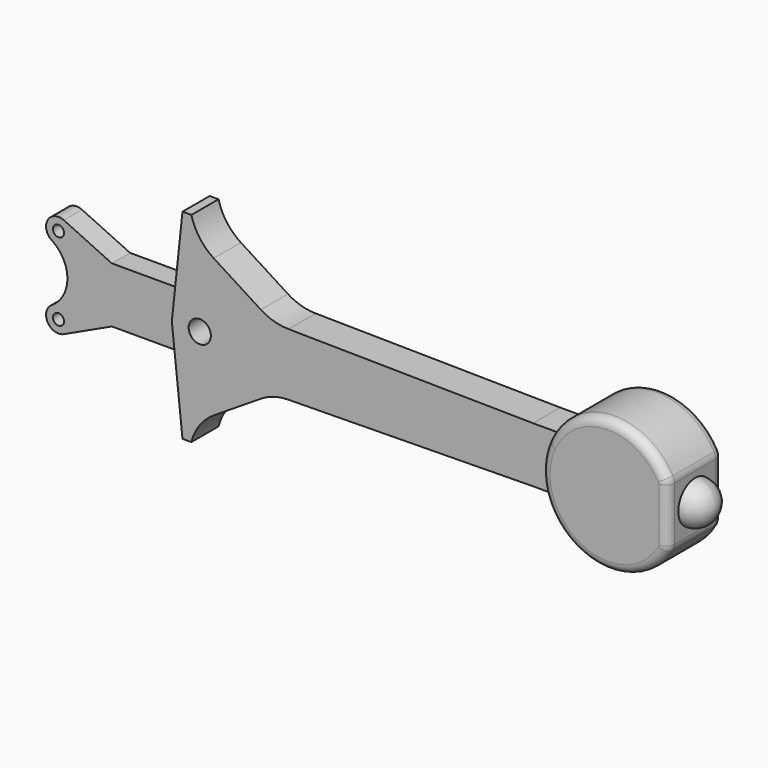
from build123d import *

# Parameters (mm, degrees)
F0_R     = 3.175
F1_DEPTH = 4.85
F3_DEPTH = 9.85
F0_R_2   = 1.5875
F4_DEPTH = 3.245
F7_R     = 3.5
F8_R     = 2.5


# Not quite as in the source:
# - ends of sketch curves that miss each other by under 0.0002 mm in the source are joined


with BuildPart() as f1:
    # F0 (on Front) → F1 (new body, symmetric)
    with BuildSketch(Plane.XZ):
        with BuildLine():
            Line((-54.121032, -0.838973), (-53.366513, -7.937497))
            Line((-53.366513, -7.937497), (-51.172903, -28.574999))
            Line((-51.172903, -28.574999), (-48.632903, -28.575001))
            ThreePointArc((-48.632903, -28.575001), (-46.273807, -23.559064), (-42.235594, -19.761986))
            Line((-42.235594, -19.761986), (-28.773587, -11.202198))
            ThreePointArc((-28.773587, -11.202198), (-24.965589, -9.479812), (-20.828003, -8.890025))
            Line((-20.828003, -8.890025), (49.021998, -7.937586))
            Line((49.021998, -7.937586), (57.104418, -7.937593))
            ThreePointArc((57.104418, -7.937593), (74.076143, -19.046968), (91.440005, -8.561076))
            Line((91.440005, -8.561076), (91.440005, 8.560861))
            ThreePointArc((91.440005, 8.560861), (74.076158, 19.046752), (57.104431, 7.937407))
            Line((57.104431, 7.937407), (49.022012, 7.937414))
            Line((49.022012, 7.937414), (-20.827987, 8.889975))
            ThreePointArc((-20.827987, 8.889975), (-24.965572, 9.479769), (-28.773568, 11.202163))
            Line((-28.773568, 11.202163), (-42.23556, 19.761974))
            ThreePointArc((-42.23556, 19.761974), (-46.273766, 23.559058), (-48.632853, 28.574999))
            Line((-48.632853, 28.574999), (-51.172853, 28.575001))
            Line((-51.172853, 28.575001), (-53.366499, 7.937503))
            Line((-53.366499, 7.937503), (-54.121031, 0.838981))
            ThreePointArc((-54.121031, 0.838981), (-54.154371, 0.420081), (-54.165495, 4e-06))
            ThreePointArc((-54.165495, 4e-06), (-54.154372, -0.420073), (-54.121032, -0.838973))
        make_face()
        with Locations((-46.227995, -3e-06)):
            Circle(F0_R, mode=Mode.SUBTRACT)
    extrude(amount=F1_DEPTH, both=True)

    # F2 (on Front) → F3 (join, symmetric)
    with BuildSketch(Plane.XZ):
        with BuildLine():
            Line((91.440005, -8.561076), (91.440005, 8.560861))
            ThreePointArc((91.440005, 8.560861), (74.076158, 19.046752), (57.104431, 7.937407))
            ThreePointArc((57.104431, 7.937407), (66.171404, -17.170725), (91.440005, -8.561076))
        make_face()
    extrude(amount=F3_DEPTH, both=True)

    # F0 (on Front) → F4 (join, symmetric)
    with BuildSketch(Plane.XZ):
        with BuildLine():
            ThreePointArc((-89.800661, 8.129989), (-85.351067, 3.1e-05), (-89.800675, -8.129919))
            ThreePointArc((-89.800675, -8.129919), (-90.999923, -12.838698), (-86.381177, -14.347999))
            Line((-86.381177, -14.347999), (-72.633744, -7.93748))
            Line((-72.633744, -7.93748), (-53.366513, -7.937497))
            Line((-53.366513, -7.937497), (-54.121032, -0.838973))
            ThreePointArc((-54.121032, -0.838973), (-54.154372, -0.420073), (-54.165495, 4e-06))
            ThreePointArc((-54.165495, 4e-06), (-54.154371, 0.420081), (-54.121031, 0.838981))
            Line((-54.121031, 0.838981), (-53.366499, 7.937503))
            Line((-53.366499, 7.937503), (-72.633731, 7.93752))
            Line((-72.633731, 7.93752), (-86.381152, 14.348062))
            ThreePointArc((-86.381152, 14.348062), (-90.9999, 12.83877), (-89.800661, 8.129989))
        make_face()
        with Locations((-87.884005, -11.125167)):
            Circle(F0_R_2, mode=Mode.SUBTRACT)
        with Locations((-87.883985, 11.125233)):
            Circle(F0_R_2, mode=Mode.SUBTRACT)
    extrude(amount=F4_DEPTH, both=True)

    # F5 (on Front) → F6 (revolve)
    with BuildSketch(Plane.XZ):
        with BuildLine():
            Line((90.440005, 0), (97.440005, 0))
            ThreePointArc((97.440005, 0), (95.682646, 4.242641), (91.440005, 6))
            Line((91.440005, 6), (90.440005, 6))
            Line((90.440005, 6), (90.440005, 0))
        make_face()
    revolve(axis=Axis((87.626113, 0, 0), (1, 0, 0)))

    # F7
    f7_edges = [f1.edges().sort_by_distance(p)[0] for p in [
        (91.440005, 0, -8.561076),
        (91.440005, 0, 8.560861),
    ]]
    fillet(f7_edges, radius=F7_R)

    # F8
    f8_edges = [f1.edges().sort_by_distance(p)[0] for p in [
        (91.440005, -9.85, -0.000108),
        (91.323733, -9.85, -8.580203),
        (91.323733, -9.85, 8.579988),
        (55.372005, -9.85, -0.000108),
        (91.440005, 9.85, -0.000108),
        (91.323733, 9.85, -8.580203),
        (91.323733, 9.85, 8.579988),
        (55.372005, 9.85, -0.000108),
    ]]
    fillet(f8_edges, radius=F8_R)


solid = f1.part
